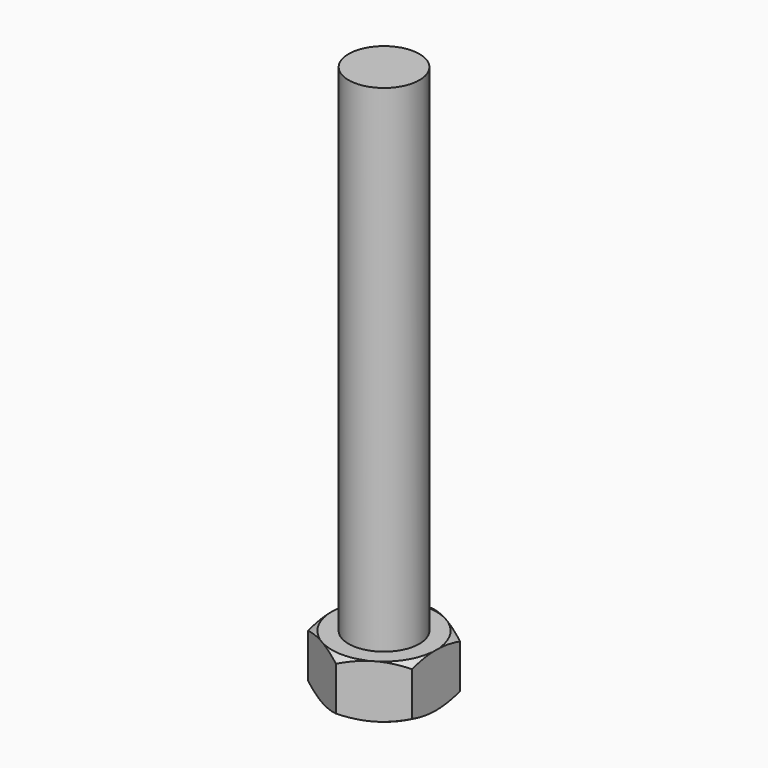
from build123d import *

# Parameters (mm, degrees)
F0_R     = 12.7
F1_DEPTH = 177.8
F2_R     = 12.7
F3_DEPTH = 19.05


with BuildPart() as f1:
    # F0 (on Top) → F1 (new body)
    with BuildSketch(Plane.XY):
        Circle(F0_R)
    extrude(amount=F1_DEPTH)

    # F2 (on face) → F3 (join)
    with BuildSketch(Plane(origin=(0, 0, 0), x_dir=(1, 0, 0), z_dir=(0, 0, -1))):
        Polygon((0, -21.5293582698), (18.6449711888, -10.7646791349), (18.6449711888, 10.7646791349), (0, 21.5293582698), (-18.6449711888, 10.7646791349), (-18.6449711888, -10.7646791349), align=None)
        Circle(F2_R, mode=Mode.SUBTRACT)
        Circle(F2_R)
    extrude(amount=F3_DEPTH)

    # F4 (on Front) → F5 (revolve, cut)
    with BuildSketch(Plane.XZ):
        Polygon((31.3791224592, -11.6979343361), (18.6449711888, -19.05), (31.3791224592, -19.05), align=None)
        Polygon((18.6449711888, 0), (31.3791224592, -7.3520656639), (31.3791224592, 0), align=None)
    revolve(axis=Axis((0, 0, -9.525), (0, 0, -1)), mode=Mode.SUBTRACT)


solid = f1.part
